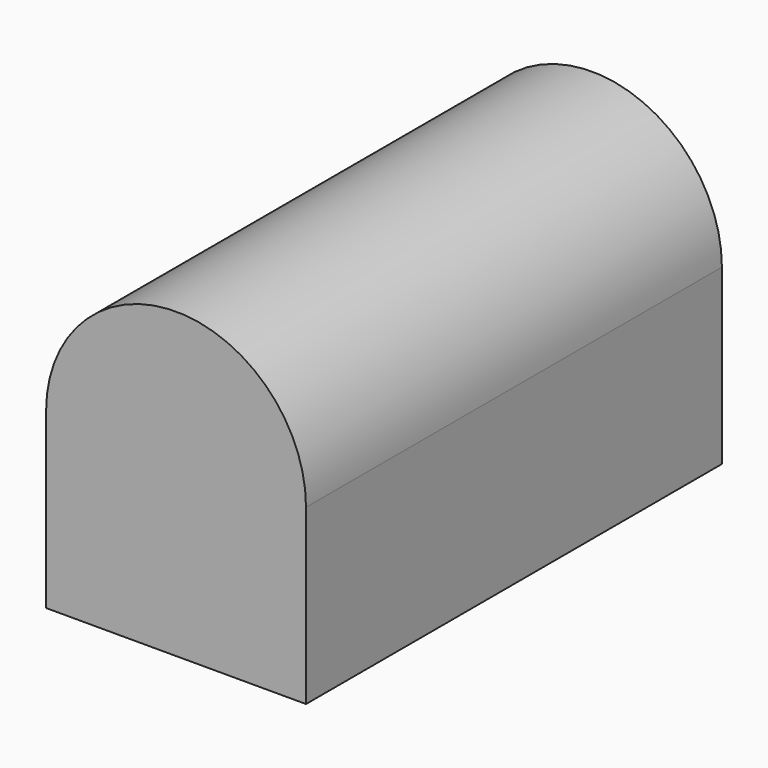
from build123d import *

# Parameters (mm, degrees)
F1_R     = 12.7
F2_DEPTH = 76.2


# Not quite as in the source:
# - a feature of the source that left no trace in its solid (it failed there, or was rolled back) is left out


with BuildPart() as f2:
    # F1 (on face) → F2 (new body)
    with BuildSketch(Plane.XZ):
        with Locations((0, 3.175)):
            Circle(F1_R)
    extrude(amount=F2_DEPTH)


with BuildPart() as f2b:
    # F0 (on Front) → F2, piece 2 (new body)
    with BuildSketch(Plane.XZ):
        with BuildLine():
            Line((-19.05, 3.175), (-19.05, -22.225))
            Line((-19.05, -22.225), (19.05, -22.225))
            Line((19.05, -22.225), (19.05, 3.175))
            ThreePointArc((19.05, 3.175), (0, -15.875), (-19.05, 3.175))
        make_face()
        with BuildLine():
            ThreePointArc((19.05, 3.175), (0, 22.225), (-19.05, 3.175))
            ThreePointArc((-19.05, 3.175), (0, -15.875), (19.05, 3.175))
        make_face()
    extrude(amount=F2_DEPTH)


solid = Compound([f2.part, f2b.part])
